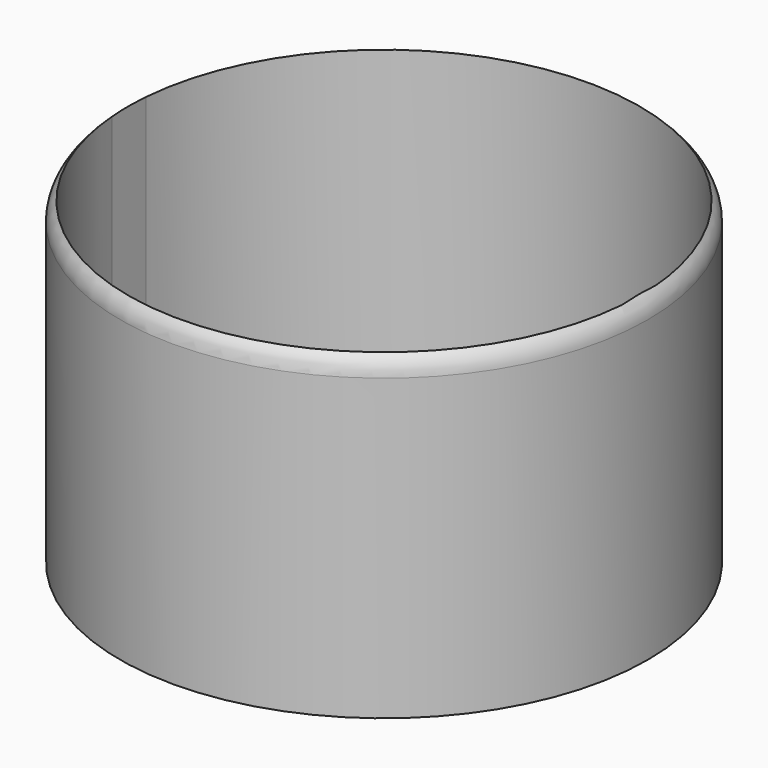
from build123d import *

# Parameters (mm, degrees)
F0_R         = 82.55
F1_DEPTH     = 101.6
F2_DEPTH     = 2.54
F3_T4_DEPTH  = 69.8204980899
F3_S5_R      = 25.3946323487
F3_T6_DEPTH  = 37
F3_T10_DEPTH = 69.8204980899
F3_S11_R     = 25.3946323487
F3_T12_DEPTH = 37
F3_T16_DEPTH = 69.8204980899
F3_S17_R     = 25.3946323487
F3_T18_DEPTH = 37
F3_T22_DEPTH = 69.8204980899
F3_S23_R     = 25.3946323487
F3_T24_DEPTH = 37


# Not quite as in the source:
# - a fillet or chamfer that OpenCascade refuses, or shapes differently, is made with other operations: its cross-section is extruded or revolved along the edge and cut away or added


with BuildPart() as f1:
    # F0 (on Top) → F1 (new body)
    with BuildSketch(Plane.XY):
        Circle(F0_R)
        with BuildLine():
            ThreePointArc((-79.7292535884, 6.6967322061), (0, 80.01), (79.7292535884, 6.6967322061))
            Line((79.7292535884, 6.6967322061), (79.7292535884, -6.6967322061))
            ThreePointArc((79.7292535884, -6.6967322061), (0, -80.01), (-79.7292535884, -6.6967322061))
            Line((-79.7292535884, -6.6967322061), (-79.7292535884, 6.6967322061))
        make_face(mode=Mode.SUBTRACT)
    extrude(amount=F1_DEPTH)

    # F0 (on Top) → F2 (join)
    with BuildSketch(Plane.XY):
        with BuildLine():
            Line((79.7292535884, -6.6967322061), (79.7292535884, 6.6967322061))
            Line((79.7292535884, 6.6967322061), (24.4957369737, 6.6967322061))
            ThreePointArc((24.4957369737, 6.6967322061), (19.4552564334, 16.321162619), (10.8538087247, 22.9582705859))
            ThreePointArc((10.8538087247, 22.9582705859), (0, 25.3946323487), (-10.8538087247, 22.9582705859))
            ThreePointArc((-10.8538087247, 22.9582705859), (-19.4552564334, 16.321162619), (-24.4957369737, 6.6967322061))
            Line((-24.4957369737, 6.6967322061), (-79.7292535884, 6.6967322061))
            Line((-79.7292535884, 6.6967322061), (-79.7292535884, -6.6967322061))
            Line((-79.7292535884, -6.6967322061), (-24.4957369737, -6.6967322061))
            ThreePointArc((-24.4957369737, -6.6967322061), (0, -25.3946323487), (24.4957369737, -6.6967322061))
            Line((24.4957369737, -6.6967322061), (79.7292535884, -6.6967322061))
        make_face()
    extrude(amount=F2_DEPTH)

    # F3: fillet of radius 7.971733183 on 5 edges, made by hand


with BuildPart() as f3_tool2:
    # F3_s3 → F3_t4 (new body)
    with BuildSketch(Plane.YZ.offset(-9.9087554985)):
        with BuildLine():
            ThreePointArc((6.6967322061, 0), (4.0437788864, 1.8774684696), (0.861939616, 2.54))
            Line((0.861939616, 2.54), (6.6967322061, 2.54))
            Line((6.6967322061, 2.54), (6.6967322061, 0))
        make_face()
    extrude(amount=-F3_T4_DEPTH)

    # F3_s5 → F3_t6 (cut, symmetric)
    with BuildSketch(Plane.XY.offset(1.3)):
        Circle(F3_S5_R)
    extrude(amount=F3_T6_DEPTH, both=True, mode=Mode.SUBTRACT)


with BuildPart() as f1_1:
    add(f1.part)

    # F3_t1: cut F3_tool2
    add(f3_tool2.part, mode=Mode.SUBTRACT)


with BuildPart() as f3_tool8:
    # F3_s9 → F3_t10 (new body)
    with BuildSketch(Plane.YZ.offset(-79.7292535884)):
        with BuildLine():
            ThreePointArc((-6.6967322061, 0), (-4.0437788864, 1.8774684696), (-0.861939616, 2.54))
            Line((-0.861939616, 2.54), (-6.6967322061, 2.54))
            Line((-6.6967322061, 2.54), (-6.6967322061, 0))
        make_face()
    extrude(amount=F3_T10_DEPTH)

    # F3_s11 → F3_t12 (cut, symmetric)
    with BuildSketch(Plane.XY.offset(1.3)):
        Circle(F3_S11_R)
    extrude(amount=F3_T12_DEPTH, both=True, mode=Mode.SUBTRACT)


with BuildPart() as f1_2:
    add(f1_1.part)

    # F3_t7: cut F3_tool8
    add(f3_tool8.part, mode=Mode.SUBTRACT)


with BuildPart() as f3_tool14:
    # F3_s15 → F3_t16 (new body)
    with BuildSketch(Plane.YZ.offset(79.7292535884)):
        with BuildLine():
            ThreePointArc((6.6967322061, 0), (4.0437788864, 1.8774684696), (0.861939616, 2.54))
            Line((0.861939616, 2.54), (6.6967322061, 2.54))
            Line((6.6967322061, 2.54), (6.6967322061, 0))
        make_face()
    extrude(amount=-F3_T16_DEPTH)

    # F3_s17 → F3_t18 (cut, symmetric)
    with BuildSketch(Plane.XY.offset(1.3)):
        Circle(F3_S17_R)
    extrude(amount=F3_T18_DEPTH, both=True, mode=Mode.SUBTRACT)


with BuildPart() as f1_3:
    add(f1_2.part)

    # F3_t13: cut F3_tool14
    add(f3_tool14.part, mode=Mode.SUBTRACT)


with BuildPart() as f3_tool20:
    # F3_s21 → F3_t22 (new body)
    with BuildSketch(Plane.YZ.offset(9.9087554985)):
        with BuildLine():
            ThreePointArc((-6.6967322061, 0), (-4.0437788864, 1.8774684696), (-0.861939616, 2.54))
            Line((-0.861939616, 2.54), (-6.6967322061, 2.54))
            Line((-6.6967322061, 2.54), (-6.6967322061, 0))
        make_face()
    extrude(amount=F3_T22_DEPTH)

    # F3_s23 → F3_t24 (cut, symmetric)
    with BuildSketch(Plane.XY.offset(1.3)):
        Circle(F3_S23_R)
    extrude(amount=F3_T24_DEPTH, both=True, mode=Mode.SUBTRACT)


with BuildPart() as f1_4:
    add(f1_3.part)

    # F3_t19: cut F3_tool20
    add(f3_tool20.part, mode=Mode.SUBTRACT)

    # F3_s25 → F3_t26 (revolve, cut)
    with BuildSketch(Plane.XZ):
        with BuildLine():
            ThreePointArc((82.55, 93.628266817), (80.2151334085, 99.2651334085), (74.578266817, 101.6))
            Line((74.578266817, 101.6), (82.55, 101.6))
            Line((82.55, 101.6), (82.55, 93.628266817))
        make_face()
    revolve(axis=Axis((0, 0, 101.6), (0, 0, 1)), mode=Mode.SUBTRACT)


solid = f1_4.part
